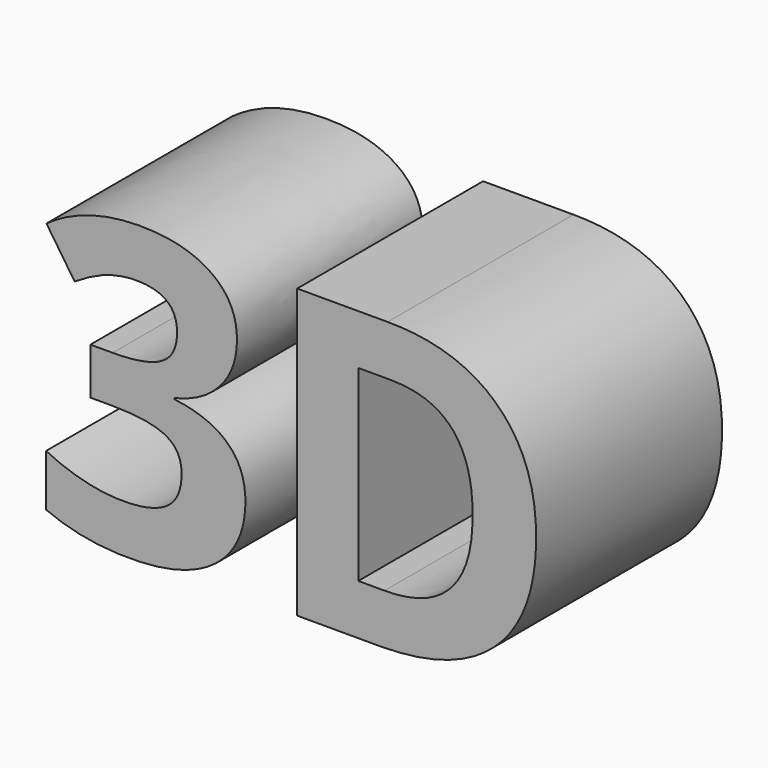
from build123d import *

# Parameters (mm, degrees)
F0_TEXT_SIZE = 176.3888888889
F1_DEPTH     = 101.6


# Not quite as in the source:
# - Text() gives the source's letters only with a copy of the font that has no kerning and outlines rounded to 1/6400 em; it was checked with that copy


with BuildPart() as f1:
    # F0 (on Front) → F1 (new body)
    with BuildSketch(Plane.XZ):
        with Locations((0, 0)):
            Text('3D', F0_TEXT_SIZE, font='Open Sans', font_style=FontStyle.BOLD, text_align=(TextAlign.LEFT, TextAlign.BOTTOM))
    extrude(amount=F1_DEPTH)


solid = f1.part
